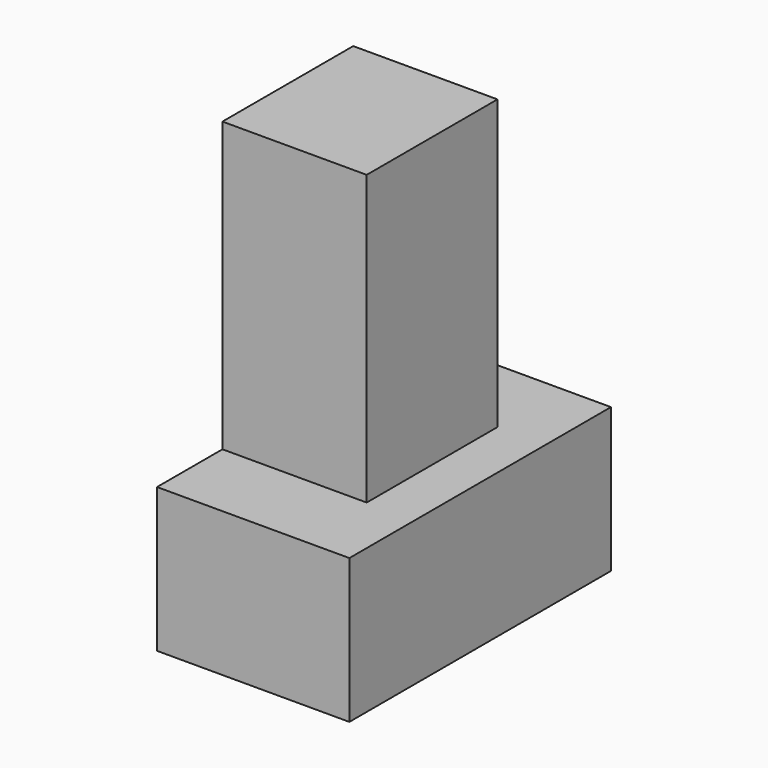
from build123d import *

# Parameters (mm, degrees)
F0_W     = 50.8
F0_H     = 86.36
F1_DEPTH = 25.4
F2_W     = 38.1
F2_H     = 76.2
F3_DEPTH = 101.6
F4_W     = 50.8
F4_H     = 86.36
F4_W_2   = 38.1
F4_H_2   = 76.2
F5_DEPTH = 12.7
F6_W     = 12.7
F6_H     = 21.59
F7_DEPTH = 76.2


with BuildPart() as f1:
    # F0 (on Top) → F1 (new body)
    with BuildSketch(Plane.XY):
        Rectangle(F0_W, F0_H)
    extrude(amount=F1_DEPTH)

    # F2 (on face) → F3 (cut)
    with BuildSketch(Plane.XY.offset(25.4)):
        Rectangle(F2_W, F2_H)
    extrude(amount=-F3_DEPTH, mode=Mode.SUBTRACT)

    # F4 (on face) → F5 (join)
    with BuildSketch(Plane.XY.offset(25.4)):
        Rectangle(F4_W, F4_H)
        Rectangle(F4_W_2, F4_H_2, mode=Mode.SUBTRACT)
        Rectangle(F4_W_2, F4_H_2)
    extrude(amount=F5_DEPTH)

    # F6 (on face) → F7 (join)
    with BuildSketch(Plane.XY.offset(38.1)):
        with Locations((-19.05, 10.795)):
            Rectangle(F6_W, F6_H)
        with Locations((-6.35, 10.795)):
            Rectangle(F6_W, F6_H)
        with Locations((-19.05, -10.795)):
            Rectangle(F6_W, F6_H)
        Polygon((12.7, 21.59), (0, 21.59), (0, 0), (0, -21.59), (12.7, -21.59), (12.7, 0), align=None)
        with Locations((-6.35, -10.795)):
            Rectangle(F6_W, F6_H)
    extrude(amount=F7_DEPTH)


solid = f1.part
